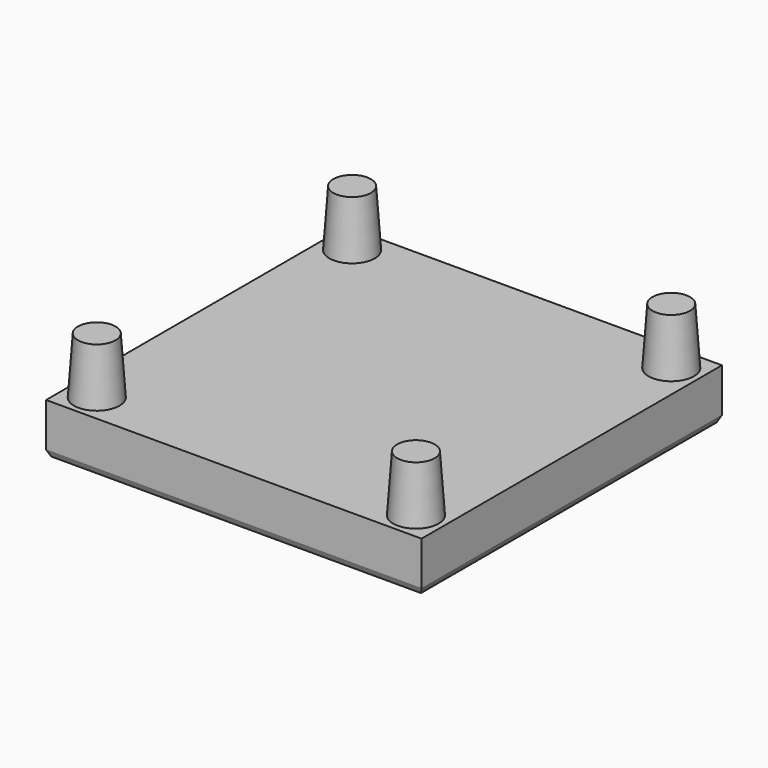
from build123d import *

# Parameters (mm, degrees)
F0_W         = 30
F0_H         = 30
F1_DEPTH     = 4
F2_R         = 1.5
F3_DEPTH     = 4.5
F4_C1_SIZE2  = 0.2331538291
F4_C1_SIZE   = 0.5
F4_C2_SIZE2  = 0.2331538291
F4_C2_SIZE   = 0.5
F4_C3_SIZE2  = 0.5
F4_C3_SIZE   = 0.2331538291
F4_C4_SIZE2  = 0.2331538291
F4_C4_SIZE   = 0.5
F6_TEXT_SIZE = 4.1666666667
F7_DEPTH     = 0.5


# Not quite as in the source:
# - a fillet or chamfer that OpenCascade refuses, or shapes differently, is made with other operations: its cross-section is extruded or revolved along the edge and cut away or added
# - Text() gives the source's letters only with a copy of the font that has no kerning and outlines rounded to 1/6400 em; it was checked with that copy


with BuildPart() as f1:
    # F0 (on Top) → F1 (new body)
    with BuildSketch(Plane.XY):
        Rectangle(F0_W, F0_H)
    extrude(amount=F1_DEPTH)

    # F2 (on face) → F3 (join)
    with BuildSketch(Plane.XY.offset(4)):
        with Locations((-12.75, 12.75)):
            Circle(F2_R)
        with Locations((-12.75, -12.75)):
            Circle(F2_R)
        with Locations((12.75, -12.75)):
            Circle(F2_R)
        with Locations((12.75, 12.75)):
            Circle(F2_R)
    extrude(amount=F3_DEPTH)

    # F4: chamfer of 0.5 x 0.2331538291 on 4 edges, made by hand

    # F4_c1
    f4_c1_edges = [f1.edges().sort_by_distance(p)[0] for p in [
        (-15, 0, 0),
    ]]
    f4_c1_side = f1.faces().sort_by_distance((-15, 0, 0.0046630766))[0]
    chamfer(f4_c1_edges, length=F4_C1_SIZE, length2=F4_C1_SIZE2, reference=f4_c1_side)

    # F4_c2
    f4_c2_edges = [f1.edges().sort_by_distance(p)[0] for p in [
        (0.1165769145, 15, 0),
    ]]
    f4_c2_side = f1.faces().sort_by_distance((0.1165769145, 15, 0.0046630766))[0]
    chamfer(f4_c2_edges, length=F4_C2_SIZE, length2=F4_C2_SIZE2, reference=f4_c2_side)

    # F4_c3
    f4_c3_edges = [f1.edges().sort_by_distance(p)[0] for p in [
        (0.1165769145, -15, 0),
    ]]
    f4_c3_side = f1.faces().sort_by_distance((0.1165769145, -14.9953369234, 0))[0]
    chamfer(f4_c3_edges, length=F4_C3_SIZE, length2=F4_C3_SIZE2, reference=f4_c3_side)

    # F4_c4
    f4_c4_edges = [f1.edges().sort_by_distance(p)[0] for p in [
        (15, 0, 0),
    ]]
    f4_c4_side = f1.faces().sort_by_distance((15, 0, 0.0046630766))[0]
    chamfer(f4_c4_edges, length=F4_C4_SIZE, length2=F4_C4_SIZE2, reference=f4_c4_side)

    # F5: chamfer of 0.315 x 4.5047098709 on 4 edges, made by hand


with BuildPart() as f5_tool2:
    # F5_s3 → F5_t4 (revolve)
    with BuildSketch(Plane.XZ.offset(-12.75)):
        Polygon((14.565, 4), (14.25, 8.5047098709), (14.25, 4), align=None)
    revolve(axis=Axis((12.75, 12.75, 4), (0, 0, 1)))

    split(bisect_by=Plane.XY.offset(8.5), keep=Keep.BOTTOM)


with BuildPart() as f1_1:
    add(f1.part)

    # F5_t1: union F5_tool2
    add(f5_tool2.part)


with BuildPart() as f5_tool7:
    # F5_s8 → F5_t9 (revolve)
    with BuildSketch(Plane.XZ.offset(-12.75)):
        Polygon((-10.935, 4), (-11.25, 8.5047098709), (-11.25, 4), align=None)
    revolve(axis=Axis((-12.75, 12.75, 4), (0, 0, 1)))

    split(bisect_by=Plane.XY.offset(8.5), keep=Keep.BOTTOM)


with BuildPart() as f1_2:
    add(f1_1.part)

    # F5_t6: union F5_tool7
    add(f5_tool7.part)


with BuildPart() as f5_tool12:
    # F5_s13 → F5_t14 (revolve)
    with BuildSketch(Plane.XZ.offset(12.75)):
        Polygon((14.565, 4), (14.25, 8.5047098709), (14.25, 4), align=None)
    revolve(axis=Axis((12.75, -12.75, 4), (0, 0, 1)))

    split(bisect_by=Plane.XY.offset(8.5), keep=Keep.BOTTOM)


with BuildPart() as f1_3:
    add(f1_2.part)

    # F5_t11: union F5_tool12
    add(f5_tool12.part)


with BuildPart() as f5_tool17:
    # F5_s18 → F5_t19 (revolve)
    with BuildSketch(Plane.XZ.offset(12.75)):
        Polygon((-10.935, 4), (-11.25, 8.5047098709), (-11.25, 4), align=None)
    revolve(axis=Axis((-12.75, -12.75, 4), (0, 0, 1)))

    split(bisect_by=Plane.XY.offset(8.5), keep=Keep.BOTTOM)


with BuildPart() as f1_4:
    add(f1_3.part)

    # F5_t16: union F5_tool17
    add(f5_tool17.part)

    # F6 (on face) → F7 (cut)
    with BuildSketch(Plane(origin=(0, 0, 0), x_dir=(1, 0, 0), z_dir=(0, 0, -1))):
        with BuildLine():
            Line((0.6243489583, 11.7470194083), (1.3404947917, 11.7470194083))
            Line((1.3404947917, 11.7470194083), (1.3404947917, 12.2515766999))
            add(Edge.make_bspline(
                [(1.3404947917, 12.2515766999), (1.3404947917, 12.3778787833), (1.3509114583, 12.6177876374)],
                knots=[0, 0, 0, 1, 1, 1], degree=2))
            add(Edge.make_bspline(
                [(1.3509114583, 12.6177876374), (1.361328125, 12.8576964916), (1.3671875, 12.8967589916)],
                knots=[0, 0, 0, 1, 1, 1], degree=2))
            Line((1.3671875, 12.8967589916), (1.3509114583, 12.8967589916))
            add(Edge.make_bspline(
                [(1.3509114583, 12.8967589916), (1.275390625, 12.7294412833), (1.169921875, 12.5712381583)],
                knots=[0, 0, 0, 1, 1, 1], degree=2))
            Line((1.169921875, 12.5712381583), (0.6243489583, 11.7470194083))
        make_face()
        with Locations((0, 10.6422016999)):
            Text('4.5mm', F6_TEXT_SIZE, font='Open Sans', font_style=FontStyle.BOLD, text_align=(TextAlign.LEFT, TextAlign.BOTTOM))
    extrude(amount=-F7_DEPTH, mode=Mode.SUBTRACT)


solid = f1_4.part
